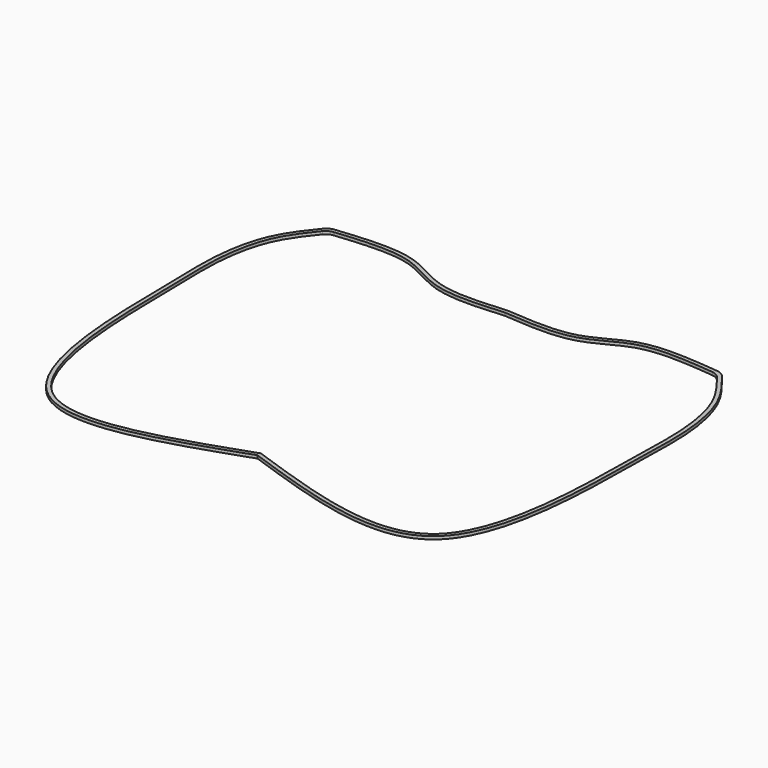
from build123d import *

# Parameters (mm, degrees)
F1_DEPTH = 1.5


# Not quite as in the source:
# - ends of sketch curves that miss each other by under 0.0002 mm in the source are joined
# - the dataset's text gives a spline's control points without its knots; the knots are read off the source's solid


with BuildPart() as f1:
    # F0 (on Top) → F1 (new body)
    with BuildSketch(Plane.XY):
        with BuildLine():
            ThreePointArc((-97.5433771491, 90.2515123967), (-99.7732185843, 89.5689168848), (-101.5743989316, 88.0877420756))
            add(Edge.make_bspline(
                [(-101.5743989316, 88.0877420756), (-106.3054813718, 82.3203643785), (-116.1760437519, 69.6730648855), (-121.240157982, 41.0931939899), (-119.3774634779, 10.4721198263), (-120.1700038549, -122.6853280032), (-40.0631451339, -94.7572371489), (0, -80.7898044586)],
                knots=[0.0137559145, 0.0137559145, 0.0137559145, 0.0137559145, 0.1380458981, 0.2812522394, 0.4452381836, 0.7225518074, 1, 1, 1, 1], degree=3))
            add(Edge.make_bspline(
                [(101.5743989316, 88.0877420756), (106.3054813718, 82.3203643785), (116.1760437519, 69.6730648855), (121.240157982, 41.0931939899), (119.3774634779, 10.4721198263), (120.1700038549, -122.6853280032), (40.0631451339, -94.7572371489), (0, -80.7898044586)],
                knots=[0.0137559145, 0.0137559145, 0.0137559145, 0.0137559145, 0.1380458981, 0.2812522394, 0.4452381836, 0.7225518074, 1, 1, 1, 1], degree=3))
            ThreePointArc((101.5743989316, 88.0877420756), (99.7732185843, 89.5689168848), (97.5433771491, 90.2515123967))
            add(Edge.make_bspline(
                [(0, 78.7864923477), (12.5380509122, 77.8055720507), (35.8479653614, 75.9819099547), (57.2853322785, 93.9733043016), (83.2041603529, 91.7117365002), (97.5433771491, 90.2515123967)],
                knots=[0, 0, 0, 0, 0.3389038678, 0.6300676412, 0.9800250153, 0.9800250153, 0.9800250153, 0.9800250153], degree=3))
            add(Edge.make_bspline(
                [(0, 78.7864923477), (-12.5380509122, 77.8055720507), (-35.8479653614, 75.9819099547), (-57.2853322785, 93.9733043016), (-83.2041603529, 91.7117365002), (-97.5433771491, 90.2515123967)],
                knots=[0, 0, 0, 0, 0.3389038678, 0.6300676412, 0.9800250153, 0.9800250153, 0.9800250153, 0.9800250153], degree=3))
        make_face()
        with BuildLine():
            add(Edge.make_bspline(
                [(3.6e-09, 76.7803811119), (-2.2605256906, 76.603537871), (-6.8454032547, 76.2458028771), (-13.6872644381, 75.8480454546), (-20.4206024218, 75.7402780253), (-25.82081743, 76.0229515695), (-29.9692134435, 76.5541570086), (-32.4811570004, 77.0317119747), (-34.4352331955, 77.511896811), (-36.3529571842, 78.063306066), (-38.6470951091, 78.8760188375), (-41.262837749, 79.9939719726), (-44.6109236616, 81.6100788155), (-47.8168712229, 83.318435944), (-51.0159533846, 84.9457361395), (-53.4451613803, 86.0865561834), (-55.9386041827, 87.1100262238), (-58.0988160289, 87.8357610064), (-59.8977106305, 88.3221357079), (-61.7617828736, 88.7497791172), (-64.2024185374, 89.1771352774), (-67.2944348127, 89.5308478409), (-71.6122099465, 89.8083066635), (-77.3344624932, 89.8270103679), (-84.5924099075, 89.4482697102), (-91.0460361437, 88.8911221518), (-95.0520685016, 88.4936657834), (-96.5154205214, 88.3455929083)],
                knots=[0.0014054227, 0.0014054227, 0.0014054227, 0.0014054227, 0.0625, 0.125, 0.1875, 0.25, 0.28125, 0.3125, 0.328125, 0.34375, 0.375, 0.40625, 0.4375, 0.5, 0.53125, 0.5625, 0.59375, 0.625, 0.640625, 0.65625, 0.6875, 0.71875, 0.75, 0.8125, 0.875, 0.9375, 0.9732985278, 0.9732985278, 0.9732985278, 0.9732985278], degree=3))
            add(Edge.make_bspline(
                [(3.6e-09, 76.7803811119), (2.2605256906, 76.603537871), (6.8454032547, 76.2458028771), (13.6872644381, 75.8480454546), (20.4206024218, 75.7402780253), (25.82081743, 76.0229515695), (29.9692134435, 76.5541570086), (32.4811570004, 77.0317119747), (34.4352331955, 77.511896811), (36.3529571842, 78.063306066), (38.6470951091, 78.8760188375), (41.262837749, 79.9939719726), (44.6109236616, 81.6100788155), (47.8168712229, 83.318435944), (51.0159533846, 84.9457361395), (53.4451613803, 86.0865561834), (55.9386041827, 87.1100262238), (58.0988160289, 87.8357610064), (59.8977106305, 88.3221357079), (61.7617828736, 88.7497791172), (64.2024185374, 89.1771352774), (67.2944348127, 89.5308478409), (71.6122099465, 89.8083066635), (77.3344624932, 89.8270103679), (84.5924099075, 89.4482697102), (91.0460361437, 88.8911221518), (95.0520685016, 88.4936657834), (96.5154205214, 88.3455929083)],
                knots=[0.0014054227, 0.0014054227, 0.0014054227, 0.0014054227, 0.0625, 0.125, 0.1875, 0.25, 0.28125, 0.3125, 0.328125, 0.34375, 0.375, 0.40625, 0.4375, 0.5, 0.53125, 0.5625, 0.59375, 0.625, 0.640625, 0.65625, 0.6875, 0.71875, 0.75, 0.8125, 0.875, 0.9375, 0.9732985278, 0.9732985278, 0.9732985278, 0.9732985278], degree=3))
            ThreePointArc((96.5154205214, 88.3455929083), (98.7530369198, 87.6604880854), (100.5583815243, 86.1715187387))
            add(Edge.make_bspline(
                [(100.5583815243, 86.1715187387), (101.042251439, 85.5790711386), (102.6951266379, 83.5414360042), (105.4301200532, 80.0307146355), (108.0354459941, 76.272787655), (109.9237507035, 73.1518972384), (111.2291160882, 70.7413787114), (112.4075252461, 68.2526743183), (113.4570494445, 65.6574325992), (114.3870170871, 62.970315839), (115.4733196683, 59.291930124), (116.558157661, 54.5619863232), (117.4725894196, 48.8297590775), (118.0529092781, 43.1924890967), (118.3537556491, 37.81078446), (118.4391955989, 32.2857752093), (118.3715534763, 26.2189046742), (118.2404047936, 20.3933470027), (118.1231235455, 15.0823065926), (118.0514989377, 11.4528941455), (117.9992927668, 8.3388765561), (117.9518590972, 5.0794719552), (117.8944722452, 0.7553700964), (117.8061857466, -4.7769066407), (117.6327673938, -12.53191476), (117.255772037, -22.7873386412), (116.3694759318, -35.5119968377), (114.8737138149, -48.1692403152), (112.597054033, -60.2679249898), (109.3775399371, -71.3101186592), (105.7911790105, -79.2102953738), (102.331345062, -84.5046978255), (99.9162272894, -87.3428749443), (97.8278221585, -89.306466707), (95.6220020205, -91.0779983355), (91.4587003252, -93.6959255125), (84.6380299971, -96.1600358427), (75.1231178453, -97.2895370419), (64.4522195421, -96.7910268644), (52.828322639, -94.905927219), (40.450424677, -91.8983316589), (23.1947140728, -86.7576287337), (9.6833203927, -82.0476912173), (0.6584046142, -78.9012856305)],
                knots=[0.0184292114, 0.0184292114, 0.0184292114, 0.0184292114, 0.03125, 0.0625, 0.09375, 0.109375, 0.125, 0.140625, 0.15625, 0.171875, 0.1875, 0.21875, 0.25, 0.28125, 0.3125, 0.34375, 0.375, 0.40625, 0.421875, 0.4375, 0.4453125, 0.453125, 0.46875, 0.484375, 0.5, 0.53125, 0.5625, 0.59375, 0.625, 0.65625, 0.6875, 0.703125, 0.71875, 0.7265625, 0.734375, 0.75, 0.78125, 0.8125, 0.84375, 0.875, 0.90625, 0.9375, 1, 1, 1, 1], degree=3))
            add(Edge.make_bspline(
                [(-0.6584046142, -78.9012856305), (-0.4389364095, -78.7660229713), (0, -78.4954976529), (0.4389364095, -78.7660229713), (0.6584046142, -78.9012856305)],
                knots=[0, 0, 0, 0, 0.5, 1, 1, 1, 1], degree=3))
            add(Edge.make_bspline(
                [(-100.5583727895, 86.171511605), (-101.042251439, 85.5790711386), (-102.6951266379, 83.5414360042), (-105.4301200532, 80.0307146355), (-108.0354459941, 76.272787655), (-109.9237507035, 73.1518972384), (-111.2291160882, 70.7413787114), (-112.4075252461, 68.2526743183), (-113.4570494445, 65.6574325992), (-114.3870170871, 62.970315839), (-115.4733196683, 59.291930124), (-116.558157661, 54.5619863232), (-117.4725894196, 48.8297590775), (-118.0529092781, 43.1924890967), (-118.3537556491, 37.81078446), (-118.4391955989, 32.2857752093), (-118.3715534763, 26.2189046742), (-118.2404047936, 20.3933470027), (-118.1231235455, 15.0823065926), (-118.0514989377, 11.4528941455), (-117.9992927668, 8.3388765561), (-117.9518590972, 5.0794719552), (-117.8944722452, 0.7553700964), (-117.8061857466, -4.7769066407), (-117.6327673938, -12.53191476), (-117.255772037, -22.7873386412), (-116.3694759318, -35.5119968377), (-114.8737138149, -48.1692403152), (-112.597054033, -60.2679249898), (-109.3775399371, -71.3101186592), (-105.7911790105, -79.2102953738), (-102.331345062, -84.5046978255), (-99.9162272894, -87.3428749443), (-97.8278221585, -89.306466707), (-95.6220020205, -91.0779983355), (-91.4587003252, -93.6959255125), (-84.6380299971, -96.1600358427), (-75.1231178453, -97.2895370419), (-64.4522195421, -96.7910268644), (-52.828322639, -94.905927219), (-40.450424677, -91.8983316589), (-23.1947140728, -86.7576287337), (-9.6833203927, -82.0476912173), (-0.6584046142, -78.9012856305)],
                knots=[0.0184292114, 0.0184292114, 0.0184292114, 0.0184292114, 0.03125, 0.0625, 0.09375, 0.109375, 0.125, 0.140625, 0.15625, 0.171875, 0.1875, 0.21875, 0.25, 0.28125, 0.3125, 0.34375, 0.375, 0.40625, 0.421875, 0.4375, 0.4453125, 0.453125, 0.46875, 0.484375, 0.5, 0.53125, 0.5625, 0.59375, 0.625, 0.65625, 0.6875, 0.703125, 0.71875, 0.7265625, 0.734375, 0.75, 0.78125, 0.8125, 0.84375, 0.875, 0.90625, 0.9375, 1, 1, 1, 1], degree=3))
            ThreePointArc((-100.5583727895, 86.171511605), (-98.7530369198, 87.6604880854), (-96.5154205214, 88.3455929083))
        make_face(mode=Mode.SUBTRACT)
    extrude(amount=F1_DEPTH)


solid = f1.part
